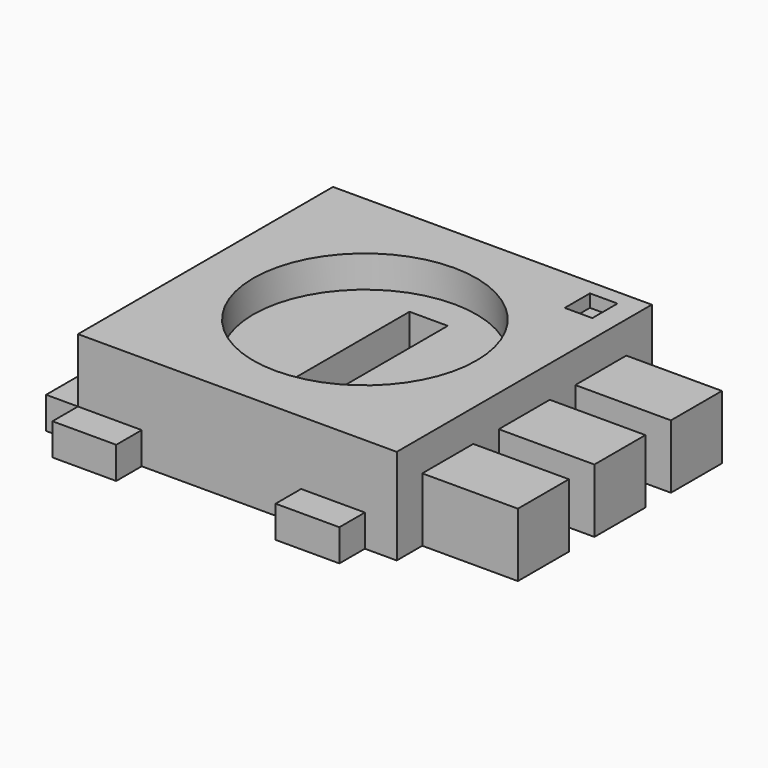
from build123d import *

# Parameters (mm, degrees)
F0_W      = 50
F0_H      = 50
F1_DEPTH  = 15
F2_W      = 6
F2_H      = 25
F3_DEPTH  = 25
F4_W      = 10
F4_H      = 10
F5_DEPTH  = 30
F6_W      = 50
F6_H      = 20
F7_DEPTH  = 30
F9_DEPTH  = 50
F10_DEPTH = 5
F11_R     = 17.5
F11_W     = 6
F11_H     = 25
F12_DEPTH = 5
F11_W_2   = 25
F11_H_2   = 5.1409158856
F11_W_3   = 5
F11_H_3   = 5
F11_H_4   = 30
F13_DEPTH = 25
F14_W     = 6
F14_H     = 6
F15_DEPTH = 20
F16_DEPTH = 15
F11_W_4   = 4.3280106038
F11_H_5   = 4.9385428429
F17_DEPTH = 2
F18_W     = 60
F18_H     = 62
F19_DEPTH = 25
F20_SCALE = 1.6
F21_DEPTH = 4
F22_DEPTH = 4


with BuildPart() as f1:
    # F0 (on Top) → F1 (new body)
    with BuildSketch(Plane.XY):
        Rectangle(F0_W, F0_H)
    extrude(amount=F1_DEPTH)

    # F2 (on face) → F3 (cut)
    with BuildSketch(Plane.XY.offset(15)):
        Rectangle(F2_W, F2_H)
    extrude(amount=-F3_DEPTH, mode=Mode.SUBTRACT)

    # F4 (on face) → F5 (join)
    with BuildSketch(Plane.YZ.offset(25)):
        with Locations((0, 7.5)):
            Rectangle(F4_W, F4_H)
        with Locations((-15, 7.5)):
            Rectangle(F4_W, F4_H)
        with Locations((15, 7.5)):
            Rectangle(F4_W, F4_H)
    extrude(amount=F5_DEPTH)

    # F6 (on face) → F7 (join)
    with BuildSketch(Plane.YZ.offset(55)):
        with Locations((0, 7.5)):
            Rectangle(F6_W, F6_H)
    extrude(amount=F7_DEPTH)

    # F8 (on face) → F9 (cut)
    with BuildSketch(Plane(origin=(0, 25, 0), x_dir=(-1, 0, 0), z_dir=(0, 1, 0))):
        Polygon((-85, -2.5), (-70, 17.5), (-85, 17.5), align=None)
    extrude(amount=-F9_DEPTH, mode=Mode.SUBTRACT)

    # F0 (on Top) → F10 (join)
    with BuildSketch(Plane.XY):
        Polygon((-25, -25), (-25, 25), (25, 25), (25, 30), (-30, 30), (-30, -30), (25, -30), (25, -25), align=None)
    extrude(amount=F10_DEPTH)

    # F11 (on face) → F12 (cut)
    with BuildSketch(Plane.XY.offset(15)):
        Circle(F11_R)
        Rectangle(F11_W, F11_H, mode=Mode.SUBTRACT)
    extrude(amount=-F12_DEPTH, mode=Mode.SUBTRACT)

    # F11 (on face) → F13 (cut)
    with BuildSketch(Plane.XY.offset(15)):
        with Locations((-2.5, -27.5704579428)):
            Rectangle(F11_W_2, F11_H_2)
        with Locations((-27.5, -27.5704579428)):
            Rectangle(F11_W_3, F11_H_2)
        with Locations((22.5, -27.5704579428)):
            Rectangle(F11_W_3, F11_H_2)
        with Locations((22.5, 27.5)):
            Rectangle(F11_W_3, F11_H_3)
        with Locations((-2.5, 27.5)):
            Rectangle(F11_W_2, F11_H_3)
        with Locations((-27.5, 27.5)):
            Rectangle(F11_W_3, F11_H_3)
        with Locations((-27.5, 0)):
            Rectangle(F11_W_3, F11_H_4)
    extrude(amount=-F13_DEPTH, mode=Mode.SUBTRACT)

    # F14 (on face) → F15 (join)
    with BuildSketch(Plane.XY.offset(17.5)):
        with Locations((67, 28)):
            Rectangle(F14_W, F14_H)
        with Locations((67, -28)):
            Rectangle(F14_W, F14_H)
    extrude(amount=-F15_DEPTH)

    # F14 (on face) → F16 (cut)
    with BuildSketch(Plane.XY.offset(17.5)):
        with Locations((67, -28)):
            Rectangle(F14_W, F14_H)
        with Locations((67, 28)):
            Rectangle(F14_W, F14_H)
    extrude(amount=-F16_DEPTH, mode=Mode.SUBTRACT)

    # F11 (on face) → F17 (cut)
    with BuildSketch(Plane.XY.offset(15)):
        with Locations((19.372981973, 20.1403833926)):
            Rectangle(F11_W_4, F11_H_5)
    extrude(amount=-F17_DEPTH, mode=Mode.SUBTRACT)

    # F18 (on face) → F19 (cut)
    with BuildSketch(Plane.XY.offset(17.5)):
        with Locations((70, 0)):
            Rectangle(F18_W, F18_H)
    extrude(amount=-F19_DEPTH, mode=Mode.SUBTRACT)


with BuildPart() as f1_1:
    # F20: moved
    add(f1.part.scale(F20_SCALE).moved(Location((0, 0, -9))))

    # F21 (add): faces of the model
    f21_faces = [f1_1.faces().sort_by_distance(p)[0] for p in [
        (52, 24, -5),
        (52, 0, -5),
        (52, -24, -5),
    ]]
    extrude(f21_faces, amount=F21_DEPTH)

    # F22 (cut): faces of the model
    f22_faces = [f1_1.faces().sort_by_distance(p)[0] for p in [
        (52, 24, 11),
        (52, 0, 11),
        (52, -24, 11),
    ]]
    extrude(f22_faces, amount=-F22_DEPTH, mode=Mode.SUBTRACT)


solid = f1_1.part
